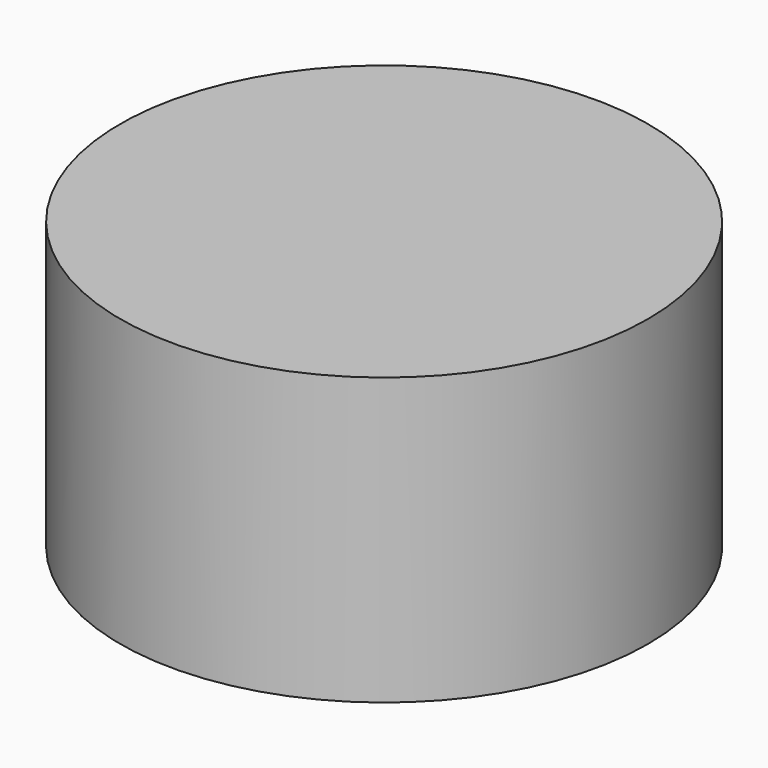
from build123d import *

# Parameters (mm, degrees)
F0_R     = 1.5
F3_DEPTH = 0.5
F4_R     = 1.55
F5_DEPTH = 1.68


# Not quite as in the source:
# - the program builds the solid bodies; features that only make, move or delete a surface that nothing else refers to are left out


with BuildPart() as f3:
    # F0 (on Top) → F3 (new body)
    with BuildSketch(Plane.XY):
        Circle(F0_R)
    extrude(amount=-F3_DEPTH)


with BuildPart() as f5:
    # F4 (on Top) → F5 (new body)
    with BuildSketch(Plane.XY):
        Circle(F4_R)
    extrude(amount=-F5_DEPTH)


solid = Compound([f3.part, f5.part])
